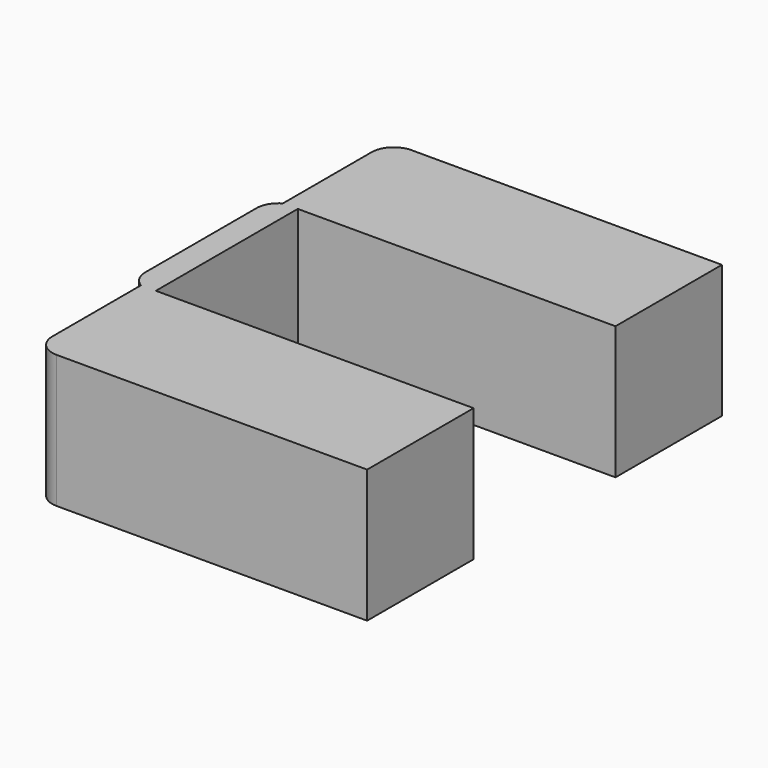
from build123d import *

# Parameters (mm, degrees)
F1_DEPTH    = 6
F2_T1_DEPTH = 10.3301270189
F2_T3_DEPTH = 11


# Not quite as in the source:
# - a fillet or chamfer that OpenCascade refuses, or shapes differently, is made with other operations: its cross-section is extruded or revolved along the edge and cut away or added


with BuildPart() as f1:
    # F0 (on Top) → F1 (new body)
    with BuildSketch(Plane.XY):
        Polygon((15, 0), (0, 0), (0, -4), (0, -6), (0.6717378856, -6), (15, -6), align=None)
        Polygon((0.6717378856, -6), (0, -6), (-0.5, -6), (-0.5, -14), (0, -14), (0.6717378856, -14), align=None)
        Polygon((15, -14), (0.6717378856, -14), (0, -14), (0, -16), (0, -20), (15, -20), align=None)
    extrude(amount=F1_DEPTH)

    # F2: fillet of radius 1 on 4 edges, made by hand

    # F2_s2 → F2_t1 (cut)
    with BuildSketch(Plane.XY.offset(-2.1650635095)):
        with BuildLine():
            ThreePointArc((0, -6), (-0.3660254038, -6.3660254038), (-0.5, -6.8660254038))
            Line((-0.5, -6.8660254038), (-0.5, -6))
            Line((-0.5, -6), (0, -6))
        make_face()
        with BuildLine():
            ThreePointArc((-0.5, -13.1339745962), (-0.3660254038, -13.6339745962), (0, -14))
            Line((0, -14), (-0.5, -14))
            Line((-0.5, -14), (-0.5, -13.1339745962))
        make_face()
    extrude(amount=F2_T1_DEPTH, mode=Mode.SUBTRACT)

    # F2_s4 → F2_t3 (cut)
    with BuildSketch(Plane.XY.offset(-2.5)):
        with BuildLine():
            ThreePointArc((1, 0), (0.2928932188, -0.2928932188), (0, -1))
            Line((0, -1), (0, 0))
            Line((0, 0), (1, 0))
        make_face()
        with BuildLine():
            ThreePointArc((0, -19), (0.2928932188, -19.7071067812), (1, -20))
            Line((1, -20), (0, -20))
            Line((0, -20), (0, -19))
        make_face()
    extrude(amount=F2_T3_DEPTH, mode=Mode.SUBTRACT)


solid = f1.part
